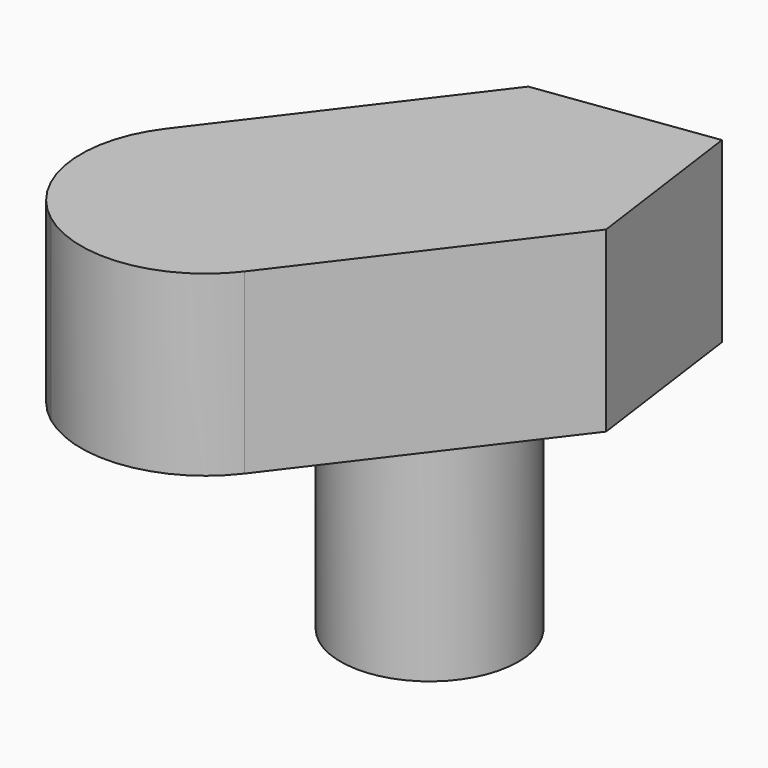
from build123d import *

# Parameters (mm, degrees)
F0_R     = 6.35
F1_DEPTH = 15.875
F3_DEPTH = 12.7
F4_SIZE  = 8.88999


# Not quite as in the source:
# - a fillet or chamfer is up to 0.001 mm smaller than in the source, because OpenCascade refuses the exact size


with BuildPart() as f1:
    # F0 (on Top) → F1 (new body)
    with BuildSketch(Plane.XY):
        Circle(F0_R)
        with BuildLine():
            Line((-1.5875, 0), (-3.556, 0))
            ThreePointArc((-3.556, 0), (0, 3.556), (3.556, 0))
            Line((3.556, 0), (1.5875, 0))
            Line((1.5875, 0), (1.5875, -1.5875))
            Line((1.5875, -1.5875), (-1.5875, -1.5875))
            Line((-1.5875, -1.5875), (-1.5875, 0))
        make_face(mode=Mode.SUBTRACT)
    extrude(amount=F1_DEPTH)

    # F2 (on face) → F3 (join)
    with BuildSketch(Plane.XY.offset(15.875)):
        with BuildLine():
            Line((17.2411291662, 7.9984802525), (10.162283151, 13.3764016998))
            Line((10.162283151, 13.3764016998), (-13.1632656924, -17.3265325287))
            ThreePointArc((-13.1632656924, -17.3265325287), (-6.5826089488, -19.0559512579), (-0.7064982299, -15.6256079608))
            Line((-0.7064982299, -15.6256079608), (17.2411291662, 7.9984802525))
        make_face()
        with BuildLine():
            Line((-13.1632656924, -17.3265325287), (10.162283151, 13.3764016998))
            Line((10.162283151, 13.3764016998), (3.0834371358, 18.7543231471))
            Line((3.0834371358, 18.7543231471), (-14.8641902603, -4.8697650662))
            ThreePointArc((-14.8641902603, -4.8697650662), (-16.5936089895, -11.4504218098), (-13.1632656924, -17.3265325287))
        make_face()
    extrude(amount=F3_DEPTH)

    # F4 (size 8.89 in the source; OpenCascade refuses exactly that, so slightly less here)
    f4_edges = [f1.edges().sort_by_distance(p)[0] for p in [
        (3.083437, 18.754323, 22.225),
        (17.241129, 7.99848, 22.225),
    ]]
    chamfer(f4_edges, length=F4_SIZE)


solid = f1.part
